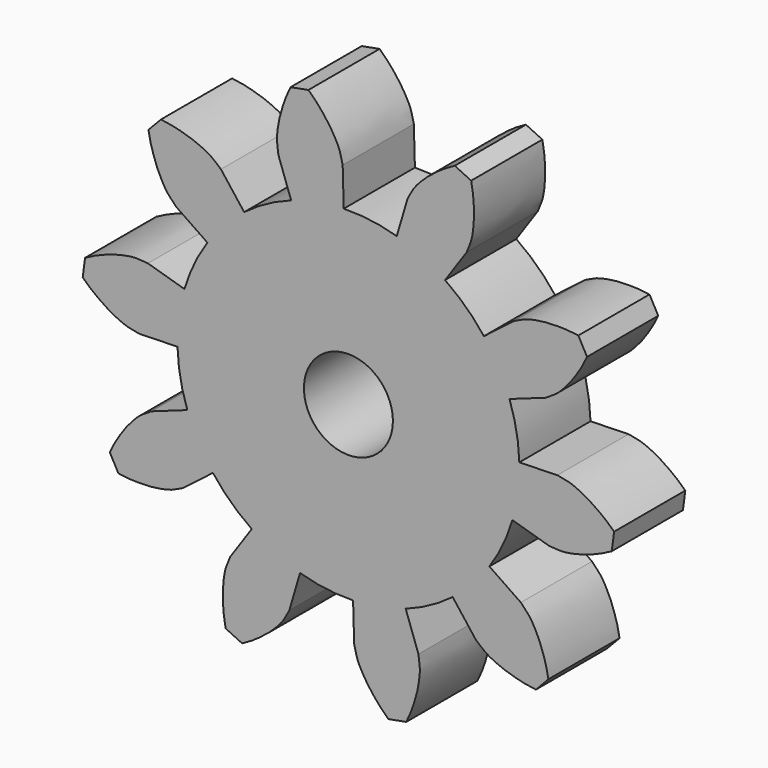
from build123d import *

# Parameters (mm, degrees)
F3_R     = 12.7
F4_DEPTH = 25.4
F5_COUNT = 10
F5_ANGLE = 324


# Not quite as in the source:
# - a variable given as a bare number and used for a length is read in inches; the dataset says mm whatever the document's units were


with BuildPart() as f4:
    # F3 (on face) → F4 (new body)
    with BuildSketch(Plane.XZ):
        with BuildLine():
            Line((-1.337879, 48.787759), (-1.635695, 59.648058))
            add(Edge.make_bspline(
                [(-1.635695, 59.648058), (-2.03818, 60.888006), (-2.256719, 62.914314), (-4.012612, 66.249422), (-5.907411, 69.293877), (-8.809916, 72.757348), (-9.698144, 73.713736), (-11.419094, 75.339527)],
                knots=[0, 0, 0, 0, 0.18993, 0.385136, 0.585303, 0.790296, 1, 1, 1, 1], degree=3))
            Line((-11.419094, 75.339527), (-16.522509, 74.387141))
            add(Edge.make_bspline(
                [(-19.987902, 56.223217), (-20.059725, 57.524872), (-20.586732, 59.493614), (-20.151911, 63.237548), (-19.482703, 66.760491), (-18.024744, 71.0377), (-17.541245, 72.250077), (-16.522509, 74.387141)],
                knots=[0, 0, 0, 0, 0.18993, 0.385136, 0.585303, 0.790296, 1, 1, 1, 1], degree=3))
            Line((-19.987902, 56.223217), (-16.348646, 45.986489))
            ThreePointArc((-16.348646, 45.986489), (-8.953495, 47.977811), (-1.337879, 48.787759))
        make_face()
        with BuildLine():
            ThreePointArc((48.8061, 0), (34.034826, 34.980938), (-1.337879, 48.787759))
            ThreePointArc((-1.337879, 48.787759), (-8.953495, 47.977811), (-16.348646, 45.986489))
            ThreePointArc((-16.348646, 45.986489), (-28.143576, -39.874485), (48.8061, 0))
        make_face()
        Circle(F3_R, mode=Mode.SUBTRACT)
    extrude(amount=F4_DEPTH)

    # F5: F4 ×10 about axis
    f5_axis = Axis((0, 0, 0), (0, -1, 0))


with BuildPart() as f4_1:
    add(f4.part)
    for i in range(1, F5_COUNT):
        add(f4.part.rotate(f5_axis, i * F5_ANGLE / (F5_COUNT - 1)))


solid = f4_1.part
